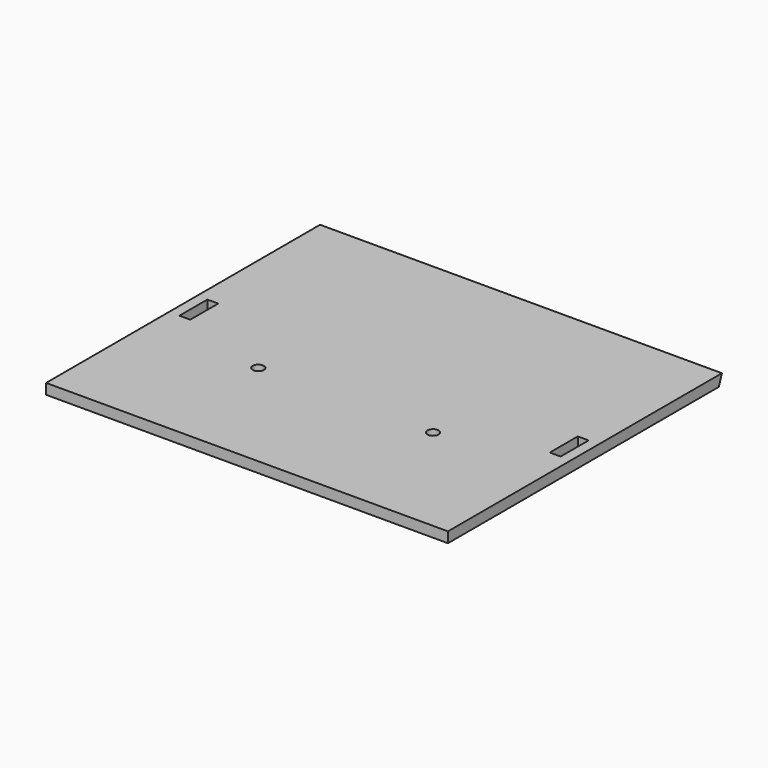
from build123d import *

# Parameters (mm, degrees)
F0_W     = 115
F0_H     = 98
F1_DEPTH = 3
F2_W     = 3.1
F2_H     = 10
F3_DEPTH = 3
F4_SIZE2 = 1.091901
F4_SIZE  = 2.99999
F8_D     = 3.2
F8_DEPTH = 5
F8_TIP   = 0.9613769904


# Not quite as in the source:
# - a fillet or chamfer is up to 0.001 mm smaller than in the source, because OpenCascade refuses the exact size
# - a pattern or mirror of a feature is missing from the dataset's text; its kind, count and spacing are read off the source's solid


with BuildPart() as f1:
    # F0 (on Top) → F1 (new body)
    with BuildSketch(Plane.XY):
        Rectangle(F0_W, F0_H)
    extrude(amount=-F1_DEPTH)

    # F2 (on face) → F3 (cut, through all)
    with BuildSketch(Plane.XY):
        with Locations((53, 0)):
            Rectangle(F2_W, F2_H)
    f3 = extrude(amount=-F3_DEPTH, mode=Mode.SUBTRACT)

    # F3_copies: F3 across plane
    add(f3.mirror(Plane(origin=(0, 0, 0), x_dir=(0, 0, -1), z_dir=(-1, 0, 0))), mode=Mode.SUBTRACT)

    # F4 (size 3 and 1.0919107028 in the source; OpenCascade refuses exactly that, so slightly less here)
    f4_edges = [f1.edges().sort_by_distance(p)[0] for p in [
        (0, 49, -3),
    ]]
    f4_side = f1.faces().sort_by_distance((0, 49, -1.5))[0]
    chamfer(f4_edges, length=F4_SIZE, length2=F4_SIZE2, reference=f4_side)

    # F8
    with Locations(Plane(origin=(0, 0, -3), x_dir=(1, 0, 0), z_dir=(0, 0, -1))):
        with Locations((25, 13.7153716188), (-25, 13.7153716188)):
            Hole(F8_D / 2, depth=F8_DEPTH)
            with Locations((0, 0, -(F8_DEPTH + F8_TIP / 2))):  # 118° drill point
                Cone(0, F8_D / 2, F8_TIP, mode=Mode.SUBTRACT)


solid = f1.part
